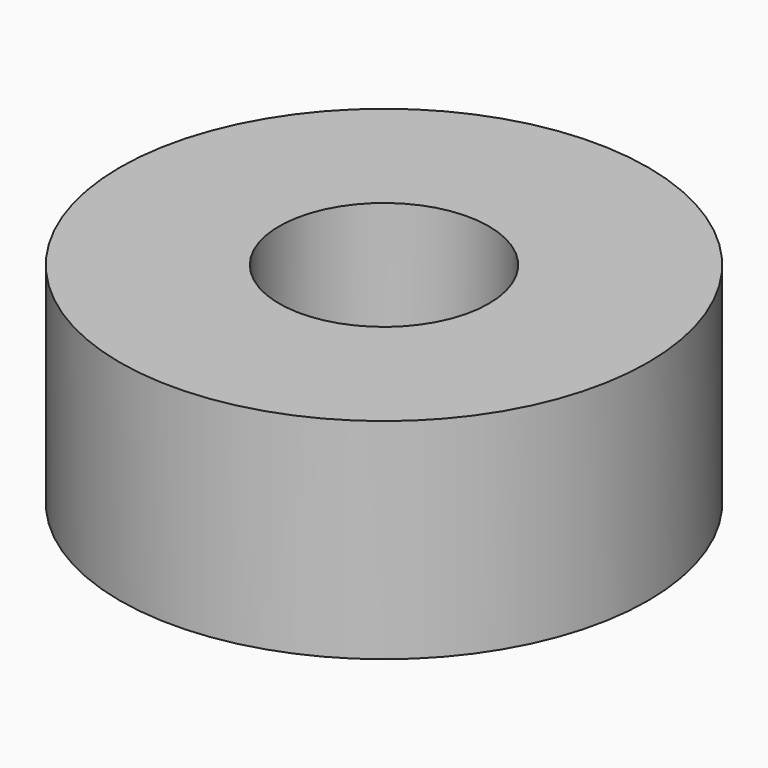
from build123d import *

# Parameters (mm, degrees)
F0_R     = 4
F0_R_2   = 1.5875
F1_DEPTH = 3.175


# Not quite as in the source:
# - a length typed as a fraction of an inch, garbled in the dataset ("3 / 203.2 mm" for 3/8 in), is restored


with BuildPart() as f1:
    # F0 (on Top) → F1 (new body)
    with BuildSketch(Plane.XY):
        Circle(F0_R)
        Circle(F0_R_2, mode=Mode.SUBTRACT)
    extrude(amount=F1_DEPTH)


solid = f1.part
